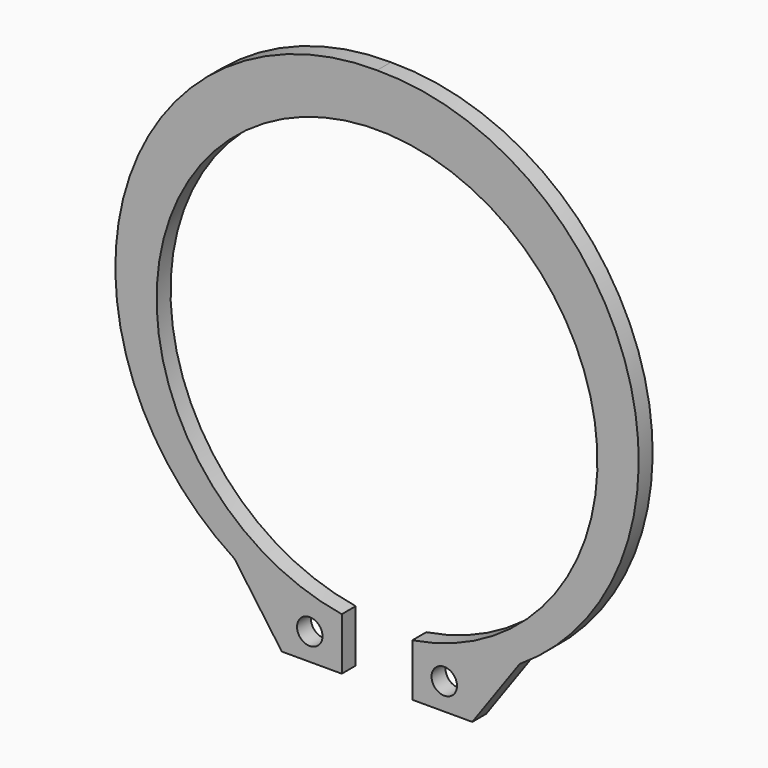
from build123d import *

# Parameters (mm, degrees)
F0_R     = 0.95
F1_DEPTH = 1.3


# Not quite as in the source:
# - ends of sketch curves that miss each other by under 0.0002 mm in the source are joined


with BuildPart() as f1:
    # F0 (on Front) → F1 (new body)
    with BuildSketch(Plane.XZ):
        with BuildLine():
            ThreePointArc((-2.631999982, -16.2380748888), (2.5478e-06, 16.45), (2.631994952, -16.2380757041))
            Line((2.631994952, -16.2380757041), (2.632, -20.148075))
            Line((2.632, -20.148075), (7.1064, -20.148075))
            Line((7.1064, -20.148075), (10.639843, -15.19527))
            ThreePointArc((10.639843, -15.19527), (18.7183878017, 6.5879564678), (-5.9926e-06, 20.349999387))
            ThreePointArc((-5.9926e-06, 20.349999387), (-18.7183877489, 6.5879566442), (-10.6398432665, -15.1952704161))
            Line((-10.6398432665, -15.1952704161), (-7.1064, -20.148075))
            Line((-7.1064, -20.148075), (-2.632, -20.148075))
            Line((-2.632, -20.148075), (-2.631999982, -16.2380748888))
        make_face()
        with Locations((-5.0192, -18.155)):
            Circle(F0_R, mode=Mode.SUBTRACT)
        with Locations((5.0192, -18.155)):
            Circle(F0_R, mode=Mode.SUBTRACT)
    extrude(amount=F1_DEPTH)


solid = f1.part
